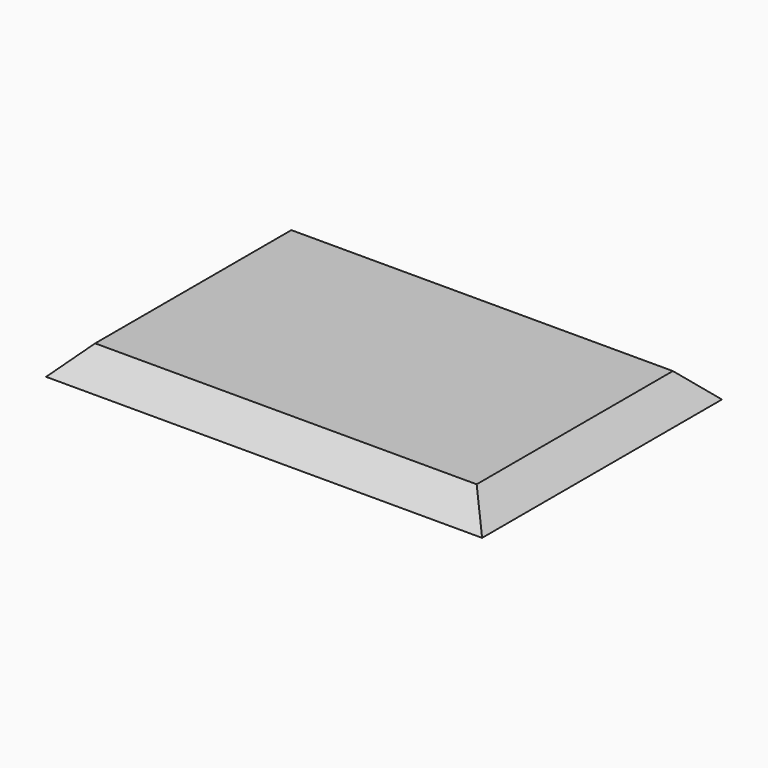
from build123d import *

# Parameters (mm, degrees)
F0_W     = 80
F0_H     = 55
F1_DEPTH = 5
F2_SIZE  = 4.99999


# Not quite as in the source:
# - a fillet or chamfer is up to 0.001 mm smaller than in the source, because OpenCascade refuses the exact size


with BuildPart() as f1:
    # F0 (on Top) → F1 (new body)
    with BuildSketch(Plane.XY):
        Rectangle(F0_W, F0_H)
    extrude(amount=F1_DEPTH)

    # F2 (size 5 in the source; OpenCascade refuses exactly that, so slightly less here)
    f2_edges = [f1.edges().sort_by_distance(p)[0] for p in [
        (0, 27.5, 5),
        (-40, 0, 5),
        (0, -27.5, 5),
        (40, 0, 5),
    ]]
    chamfer(f2_edges, length=F2_SIZE)


solid = f1.part
